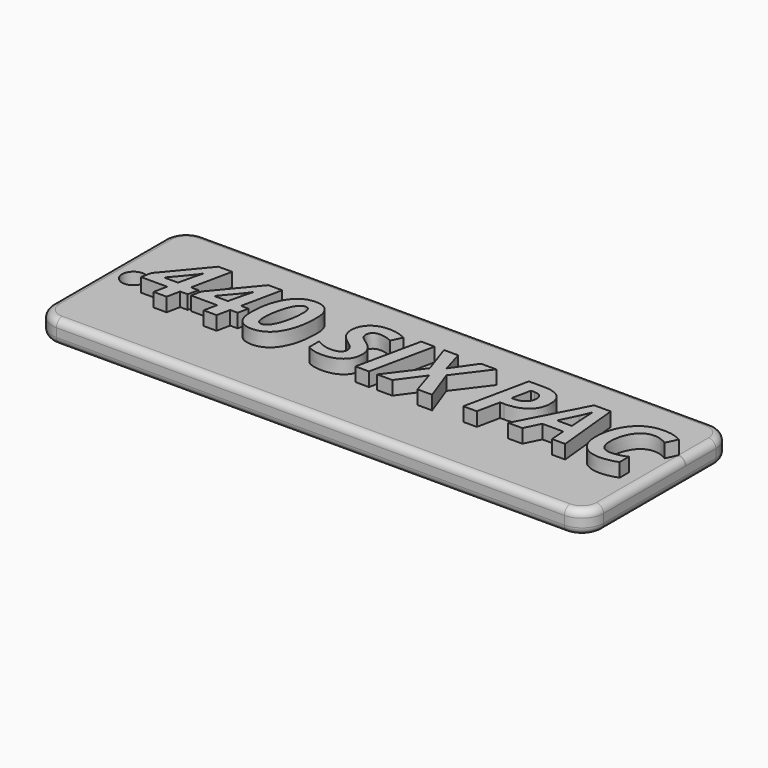
from build123d import *

# Parameters (mm, degrees)
F2_DEPTH     = 3.175
F1_TEXT_SIZE = 12.5481389996
F3_DEPTH     = 5.08
F4_R         = 1.5875
F5_DEPTH     = 3.176
F6_R         = 1
F7_R         = 1


# Not quite as in the source:
# - Text() gives the source's letters only with a copy of the font that has no kerning and outlines rounded to 1/6400 em; it was checked with that copy


with BuildPart() as f2:
    # F0 (on Top) → F2 (new body)
    with BuildSketch(Plane.XY):
        with BuildLine():
            Line((-73.2, 0), (-3, 0))
            ThreePointArc((-3, 0), (-0.8786796564, 0.8786796564), (0, 3))
            Line((0, 3), (0, 22.4))
            ThreePointArc((0, 22.4), (-0.8786796564, 24.5213203436), (-3, 25.4))
            Line((-3, 25.4), (-73.2, 25.4))
            ThreePointArc((-73.2, 25.4), (-75.3213203436, 24.5213203436), (-76.2, 22.4))
            Line((-76.2, 22.4), (-76.2, 3))
            ThreePointArc((-76.2, 3), (-75.3213203436, 0.8786796564), (-73.2, 0))
        make_face()
    extrude(amount=F2_DEPTH)

    # F1 (on face) → F3 (join)
    with BuildSketch(Plane.XY):
        with Locations((-69.85, 8.7453399203)):
            Text('440 SIX PAC', F1_TEXT_SIZE, font='Open Sans', font_style=FontStyle.BOLDITALIC, text_align=(TextAlign.LEFT, TextAlign.BOTTOM))
    extrude(amount=F3_DEPTH)

    # F4 (on face) → F5 (cut, through all)
    with BuildSketch(Plane.XY.offset(3.175)):
        with Locations((-72.7075, 12.7)):
            Circle(F4_R)
    extrude(amount=-F5_DEPTH, mode=Mode.SUBTRACT)

    # F6
    f6_edges = [f2.edges().sort_by_distance(p)[0] for p in [
        (-38.1, 0, 3.175),
    ]]
    fillet(f6_edges, radius=F6_R)

    # F7
    f7_edges = [f2.edges().sort_by_distance(p)[0] for p in [
        (-38.1, 0, 0),
    ]]
    fillet(f7_edges, radius=F7_R)


solid = f2.part
